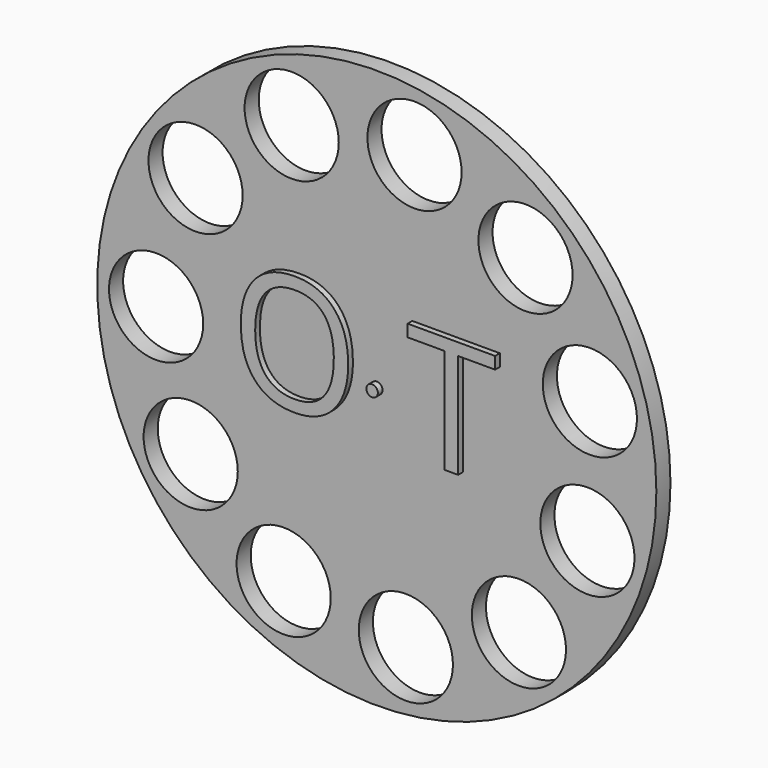
from build123d import *

# Parameters (mm, degrees)
F0_R         = 120.65
F1_DEPTH     = 7.62
F2_R         = 20.32
F3_DEPTH     = 25.4
F4_TEXT_SIZE = 70.5555555556
F5_DEPTH     = 2.54
F6_R         = 2.4837364142
F7_DEPTH     = 2.54


# Not quite as in the source:
# - Text() gives the source's letters only with a copy of the font that has no kerning and outlines rounded to 1/6400 em; it was checked with that copy


with BuildPart() as f1:
    # F0 (on Front) → F1 (new body)
    with BuildSketch(Plane.XZ):
        Circle(F0_R)
    extrude(amount=F1_DEPTH)

    # F2 (on face) → F3 (cut)
    with BuildSketch(Plane.XZ.offset(7.62)):
        with Locations((16.2726126289, 93.8496914126)):
            Circle(F2_R)
        with Locations((64.174661072, 70.3859032498)):
            Circle(F2_R)
        with Locations((91.951535803, 24.8490958279)):
            Circle(F2_R)
        with Locations((90.8924089062, -28.4803880456)):
            Circle(F2_R)
        with Locations((-36.7325271347, 87.8822163483)):
            Circle(F2_R)
        with Locations((-80.3148, -51.2064)):
            Circle(F2_R)
        with Locations((-40.19287872, -86.35447296)):
            Circle(F2_R)
        with Locations((12.5335293266, -94.4217831997)):
            Circle(F2_R)
        with Locations((61.3294225764, -72.878422228)):
            Circle(F2_R)
        with Locations((-95.25, 0)):
            Circle(F2_R)
        with Locations((-78.2183463889, 54.3548782373)):
            Circle(F2_R)
    extrude(amount=-F3_DEPTH, mode=Mode.SUBTRACT)

    # F4 (on face) → F5 (join)
    with BuildSketch(Plane.XZ.offset(7.62)):
        with Locations((-60.96, -18.5097302691)):
            Text('O', F4_TEXT_SIZE, font='Open Sans', text_align=(TextAlign.LEFT, TextAlign.BOTTOM))
        with Locations((14.7108413586, -19.882645921)):
            Text('T', F4_TEXT_SIZE, font='Open Sans', text_align=(TextAlign.LEFT, TextAlign.BOTTOM))
    extrude(amount=F5_DEPTH)

    # F6 (on face) → F7 (join)
    with BuildSketch(Plane.XZ.offset(7.62)):
        Circle(F6_R)
    extrude(amount=F7_DEPTH)


solid = f1.part
